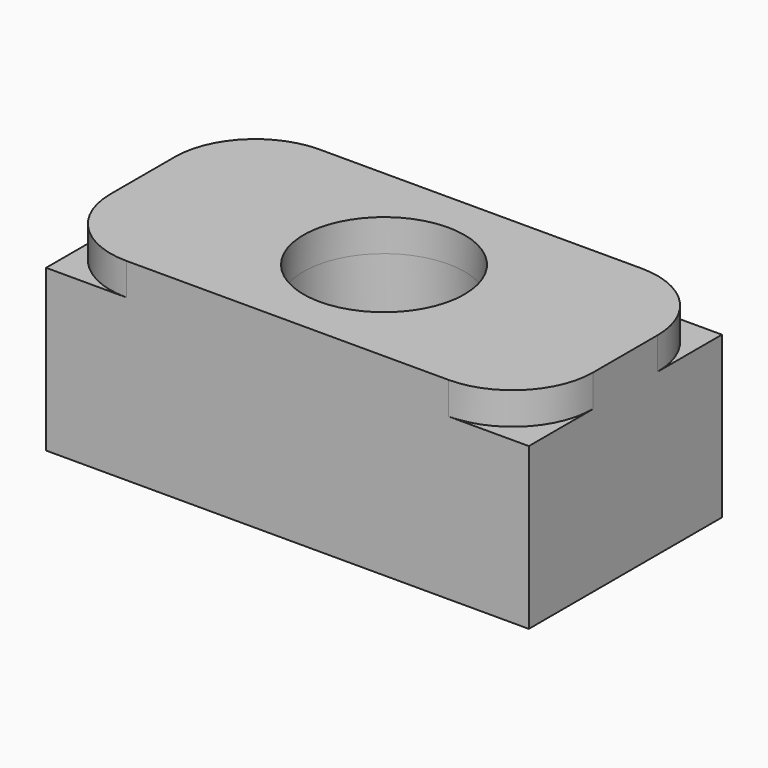
from build123d import *

# Parameters (mm, degrees)
F1_W     = 76.2
F1_H     = 38.1
F1_R     = 12.7
F2_DEPTH = 5.08
F3_R     = 12.7
F4_DEPTH = 25.4


# Not quite as in the source:
# - a variable given as a bare number and used for a length is read in inches; the dataset says mm whatever the document's units were


with BuildPart() as f2:
    # F1 (on Top) → F2 (new body)
    with BuildSketch(Plane.XY):
        Rectangle(F1_W, F1_H)
        Circle(F1_R, mode=Mode.SUBTRACT)
    extrude(amount=F2_DEPTH)

    # F3
    f3_edges = [f2.edges().sort_by_distance(p)[0] for p in [
        (38.1, -19.05, 2.54),
        (38.1, 19.05, 2.54),
        (-38.1, -19.05, 2.54),
        (-38.1, 19.05, 2.54),
    ]]
    fillet(f3_edges, radius=F3_R)

    # F1 (on Top) → F4 (join)
    with BuildSketch(Plane.XY):
        Rectangle(F1_W, F1_H)
        Circle(F1_R, mode=Mode.SUBTRACT)
    extrude(amount=-F4_DEPTH)


solid = f2.part
